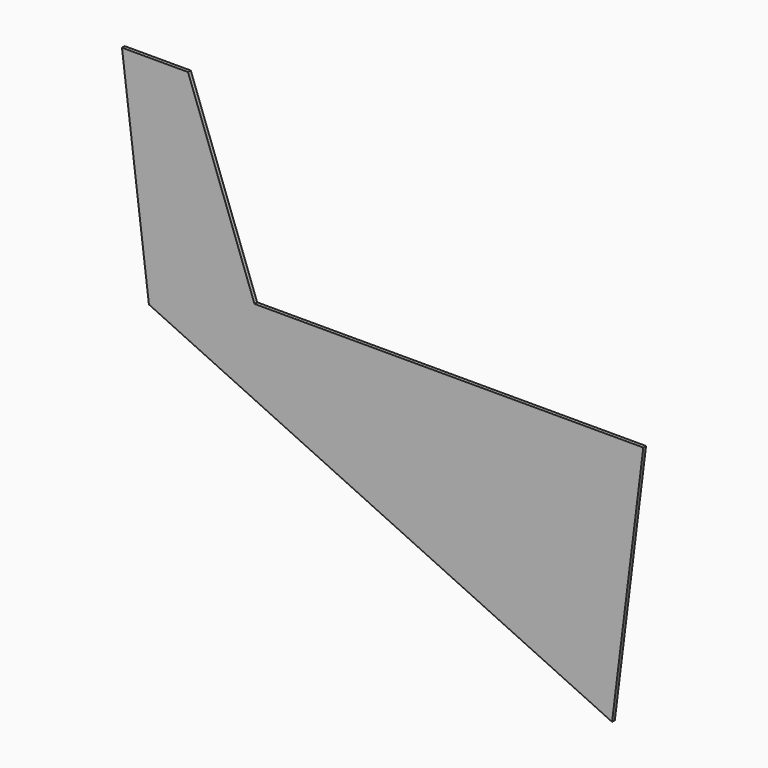
from build123d import *

# Parameters (mm, degrees)
F1_DEPTH = 4.7625


# Not quite as in the source:
# - a length typed as a fraction of an inch, garbled in the dataset ("3 / 203.2 mm" for 3/8 in), is restored


with BuildPart() as f1:
    # F0 (on Front) → F1 (new body)
    with BuildSketch(Plane.XZ):
        Polygon((-195.0059046725, 235.8100221782), (-286.9723427275, 235.8100221782), (-249.454056277, -66.6720734602), (395.2653609836, -368.5680152525), (438.7244078622, -18.1899778218), (-102.5574651689, -18.1899778218), align=None)
    extrude(amount=F1_DEPTH)


solid = f1.part
